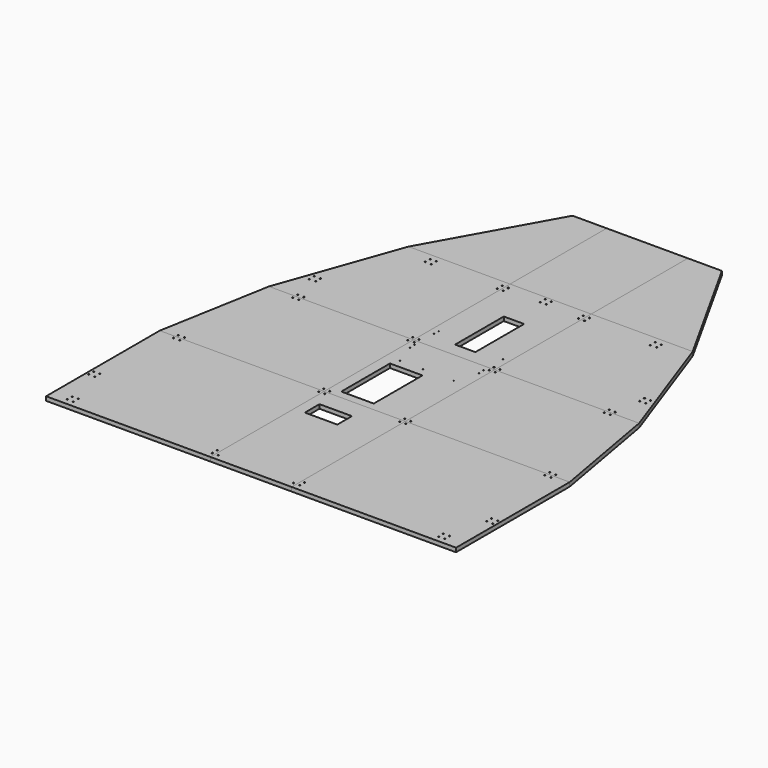
from build123d import *

# Parameters (mm, degrees)
F0_W      = 400
F0_H      = 700
F0_R      = 3
F0_W_2    = 160
F0_H_2    = 89.9538263201
F1_DEPTH  = 20
F2_R      = 3
F3_DEPTH  = 20
F4_DEPTH  = 20
F5_W      = 400
F5_H      = 550
F5_R      = 3
F5_W_2    = 160
F5_H_2    = 300
F5_R_2    = 2.05
F6_DEPTH  = 20
F7_W      = 400
F7_H      = 595
F7_R      = 3
F7_R_2    = 2.05
F7_W_2    = 100
F7_H_2    = 300
F8_DEPTH  = 20
F9_W      = 760
F9_H      = 700
F9_R      = 3
F10_DEPTH = 20
F11_W     = 400
F11_H     = 595
F12_DEPTH = 20
F14_DEPTH = 20
F16_DEPTH = 20
F17_W     = 50
F17_H     = 700
F17_R     = 3
F19_DEPTH = 20
F18_W     = 50
F18_H     = 700
F18_R     = 3
F20_DEPTH = 20
F21_R     = 3
F23_DEPTH = 20
F22_R     = 3
F24_DEPTH = 20
F26_DEPTH = 20
F28_DEPTH = 20
F30_DEPTH = 20
F32_DEPTH = 20


with BuildPart() as f1:
    # F0 (on Top) → F1 (new body)
    with BuildSketch(Plane.XY):
        Rectangle(F0_W, F0_H)
        with Locations((-185, -320)):
            Circle(F0_R, mode=Mode.SUBTRACT)
        with Locations((185, -320)):
            Circle(F0_R, mode=Mode.SUBTRACT)
        with Locations((-185, 335)):
            Circle(F0_R, mode=Mode.SUBTRACT)
        with Locations((-67.5, 210.6490433216)):
            Rectangle(F0_W_2, F0_H_2, mode=Mode.SUBTRACT)
        with Locations((185, 335)):
            Circle(F0_R, mode=Mode.SUBTRACT)
    extrude(amount=F1_DEPTH)


with BuildPart() as f3:
    # F2 (on Top) → F3 (new body)
    with BuildSketch(Plane.XY):
        Polygon((-200, 350), (-200, 900), (-812, 900), (-960, 350), align=None)
        with Locations((-930, 365)):
            Circle(F2_R, mode=Mode.SUBTRACT)
        with Locations((-900, 365)):
            Circle(F2_R, mode=Mode.SUBTRACT)
        with Locations((-215, 365)):
            Circle(F2_R, mode=Mode.SUBTRACT)
        with Locations((-782, 885)):
            Circle(F2_R, mode=Mode.SUBTRACT)
        with Locations((-752, 885)):
            Circle(F2_R, mode=Mode.SUBTRACT)
        with Locations((-215, 885)):
            Circle(F2_R, mode=Mode.SUBTRACT)
    extrude(amount=F3_DEPTH)

    # F25 (on face) → F26 (join)
    with BuildSketch(Plane(origin=(0, 0, 0), x_dir=(1, 0, 0), z_dir=(0, 0, -1))):
        Polygon((-912, -900), (-812, -900), (-960, -350), (-1010, -350), align=None)
    extrude(amount=-F26_DEPTH)


with BuildPart() as f3b:
    # F2 (on Top) → F3, piece 2 (new body)
    with BuildSketch(Plane.XY):
        Polygon((812, 900), (200, 900), (200, 350), (960, 350), align=None)
        with Locations((215, 365)):
            Circle(F2_R, mode=Mode.SUBTRACT)
        with Locations((900, 365)):
            Circle(F2_R, mode=Mode.SUBTRACT)
        with Locations((930, 365)):
            Circle(F2_R, mode=Mode.SUBTRACT)
        with Locations((215, 885)):
            Circle(F2_R, mode=Mode.SUBTRACT)
        with Locations((752, 885)):
            Circle(F2_R, mode=Mode.SUBTRACT)
        with Locations((782, 885)):
            Circle(F2_R, mode=Mode.SUBTRACT)
    extrude(amount=F3_DEPTH)

    # F27 (on face) → F28 (join)
    with BuildSketch(Plane(origin=(0, 0, 0), x_dir=(1, 0, 0), z_dir=(0, 0, -1))):
        Polygon((1010, -350), (960, -350), (812, -900), (912, -900), align=None)
    extrude(amount=-F28_DEPTH)


with BuildPart() as f4:
    # F2 (on Top) → F4 (new body)
    with BuildSketch(Plane.XY):
        Polygon((-812, 900), (-200, 900), (-200, 1495), (-600, 1495), align=None)
        with Locations((-782, 915)):
            Circle(F2_R, mode=Mode.SUBTRACT)
        with Locations((-752, 915)):
            Circle(F2_R, mode=Mode.SUBTRACT)
        with Locations((-215, 915)):
            Circle(F2_R, mode=Mode.SUBTRACT)
        with Locations((-570, 1435)):
            Circle(F2_R, mode=Mode.SUBTRACT)
        with Locations((-540, 1435)):
            Circle(F2_R, mode=Mode.SUBTRACT)
        with Locations((-570, 1465)):
            Circle(F2_R, mode=Mode.SUBTRACT)
        with Locations((-540, 1465)):
            Circle(F2_R, mode=Mode.SUBTRACT)
        with Locations((-215, 1435)):
            Circle(F2_R, mode=Mode.SUBTRACT)
        with Locations((-215, 1465)):
            Circle(F2_R, mode=Mode.SUBTRACT)
    extrude(amount=F4_DEPTH)

    # F21 (on face) → F23 (join)
    with BuildSketch(Plane(origin=(0, 0, 0), x_dir=(1, 0, 0), z_dir=(0, 0, -1))):
        Polygon((-700, -1495), (-600, -1495), (-812, -900), (-912, -900), align=None)
        with Locations((-828.415464569, -1075)):
            Circle(F21_R, mode=Mode.SUBTRACT)
        with Locations((-798.415464569, -1075)):
            Circle(F21_R, mode=Mode.SUBTRACT)
        with Locations((-828.415464569, -1045)):
            Circle(F21_R, mode=Mode.SUBTRACT)
        with Locations((-798.415464569, -1045)):
            Circle(F21_R, mode=Mode.SUBTRACT)
    extrude(amount=-F23_DEPTH)


with BuildPart() as f4b:
    # F2 (on Top) → F4, piece 2 (new body)
    with BuildSketch(Plane.XY):
        Polygon((600, 1495), (200, 1495), (200, 900), (812, 900), align=None)
        with Locations((215, 915)):
            Circle(F2_R, mode=Mode.SUBTRACT)
        with Locations((752, 915)):
            Circle(F2_R, mode=Mode.SUBTRACT)
        with Locations((782, 915)):
            Circle(F2_R, mode=Mode.SUBTRACT)
        with Locations((215, 1435)):
            Circle(F2_R, mode=Mode.SUBTRACT)
        with Locations((215, 1465)):
            Circle(F2_R, mode=Mode.SUBTRACT)
        with Locations((540, 1435)):
            Circle(F2_R, mode=Mode.SUBTRACT)
        with Locations((570, 1435)):
            Circle(F2_R, mode=Mode.SUBTRACT)
        with Locations((540, 1465)):
            Circle(F2_R, mode=Mode.SUBTRACT)
        with Locations((570, 1465)):
            Circle(F2_R, mode=Mode.SUBTRACT)
    extrude(amount=F4_DEPTH)

    # F22 (on face) → F24 (join)
    with BuildSketch(Plane(origin=(0, 0, 0), x_dir=(1, 0, 0), z_dir=(0, 0, -1))):
        Polygon((912, -900), (812, -900), (600, -1495), (700, -1495), align=None)
        with Locations((798.415464569, -1075)):
            Circle(F22_R, mode=Mode.SUBTRACT)
        with Locations((828.415464569, -1075)):
            Circle(F22_R, mode=Mode.SUBTRACT)
        with Locations((798.415464569, -1045)):
            Circle(F22_R, mode=Mode.SUBTRACT)
        with Locations((828.415464569, -1045)):
            Circle(F22_R, mode=Mode.SUBTRACT)
    extrude(amount=-F24_DEPTH)


with BuildPart() as f6:
    # F5 (on Top) → F6 (new body)
    with BuildSketch(Plane.XY):
        with Locations((0, 625)):
            Rectangle(F5_W, F5_H)
        with Locations((-185, 365)):
            Circle(F5_R, mode=Mode.SUBTRACT)
        with Locations((-67.5, 540)):
            Rectangle(F5_W_2, F5_H_2, mode=Mode.SUBTRACT)
        with Locations((185, 365)):
            Circle(F5_R, mode=Mode.SUBTRACT)
        with Locations((-132.5, 731.5)):
            Circle(F5_R_2, mode=Mode.SUBTRACT)
        with Locations((-17.5, 731.5)):
            Circle(F5_R_2, mode=Mode.SUBTRACT)
        with Locations((-170, 840)):
            Circle(F5_R_2, mode=Mode.SUBTRACT)
        with Locations((-185, 885)):
            Circle(F5_R, mode=Mode.SUBTRACT)
        with Locations((-170, 870)):
            Circle(F5_R_2, mode=Mode.SUBTRACT)
        with Locations((132.5, 731.5)):
            Circle(F5_R_2, mode=Mode.SUBTRACT)
        with Locations((170, 840)):
            Circle(F5_R_2, mode=Mode.SUBTRACT)
        with Locations((170, 870)):
            Circle(F5_R_2, mode=Mode.SUBTRACT)
        with Locations((185, 885)):
            Circle(F5_R, mode=Mode.SUBTRACT)
    extrude(amount=F6_DEPTH)


with BuildPart() as f8:
    # F7 (on Top) → F8 (new body)
    with BuildSketch(Plane.XY):
        with Locations((0, 1197.5)):
            Rectangle(F7_W, F7_H)
        with Locations((-185, 915)):
            Circle(F7_R, mode=Mode.SUBTRACT)
        with Locations((-170, 988)):
            Circle(F7_R_2, mode=Mode.SUBTRACT)
        with Locations((-170, 1018)):
            Circle(F7_R_2, mode=Mode.SUBTRACT)
        with Locations((185, 915)):
            Circle(F7_R, mode=Mode.SUBTRACT)
        with Locations((170, 988)):
            Circle(F7_R_2, mode=Mode.SUBTRACT)
        with Locations((170, 1018)):
            Circle(F7_R_2, mode=Mode.SUBTRACT)
        with Locations((0, 1119.0668344498)):
            Rectangle(F7_W_2, F7_H_2, mode=Mode.SUBTRACT)
        with Locations((-185, 1435)):
            Circle(F7_R, mode=Mode.SUBTRACT)
        with Locations((-185, 1465)):
            Circle(F7_R, mode=Mode.SUBTRACT)
        with Locations((-15, 1450)):
            Circle(F7_R, mode=Mode.SUBTRACT)
        with Locations((-15, 1480)):
            Circle(F7_R, mode=Mode.SUBTRACT)
        with Locations((15, 1450)):
            Circle(F7_R, mode=Mode.SUBTRACT)
        with Locations((15, 1480)):
            Circle(F7_R, mode=Mode.SUBTRACT)
        with Locations((185, 1435)):
            Circle(F7_R, mode=Mode.SUBTRACT)
        with Locations((185, 1465)):
            Circle(F7_R, mode=Mode.SUBTRACT)
    extrude(amount=F8_DEPTH)


with BuildPart() as f10:
    # F9 (on Top) → F10 (new body)
    with BuildSketch(Plane.XY):
        with Locations((-580, 0)):
            Rectangle(F9_W, F9_H)
        with Locations((-930, -320)):
            Circle(F9_R, mode=Mode.SUBTRACT)
        with Locations((-900, -320)):
            Circle(F9_R, mode=Mode.SUBTRACT)
        with Locations((-930, -290)):
            Circle(F9_R, mode=Mode.SUBTRACT)
        with Locations((-900, -290)):
            Circle(F9_R, mode=Mode.SUBTRACT)
        with Locations((-215, -320)):
            Circle(F9_R, mode=Mode.SUBTRACT)
        with Locations((-215, -290)):
            Circle(F9_R, mode=Mode.SUBTRACT)
        with Locations((-930, 335)):
            Circle(F9_R, mode=Mode.SUBTRACT)
        with Locations((-900, 335)):
            Circle(F9_R, mode=Mode.SUBTRACT)
        with Locations((-215, 335)):
            Circle(F9_R, mode=Mode.SUBTRACT)
    extrude(amount=F10_DEPTH)

    # F17 (on face) → F19 (join)
    with BuildSketch(Plane(origin=(0, 0, 0), x_dir=(1, 0, 0), z_dir=(0, 0, -1))):
        with Locations((-985, 0)):
            Rectangle(F17_W, F17_H)
        with Locations((-995, 75)):
            Circle(F17_R, mode=Mode.SUBTRACT)
        with Locations((-995, 105)):
            Circle(F17_R, mode=Mode.SUBTRACT)
        with Locations((-965, 75)):
            Circle(F17_R, mode=Mode.SUBTRACT)
        with Locations((-965, 105)):
            Circle(F17_R, mode=Mode.SUBTRACT)
    extrude(amount=-F19_DEPTH)


with BuildPart() as f10b:
    # F9 (on Top) → F10, piece 2 (new body)
    with BuildSketch(Plane.XY):
        with Locations((580, 0)):
            Rectangle(F9_W, F9_H)
        with Locations((215, -320)):
            Circle(F9_R, mode=Mode.SUBTRACT)
        with Locations((215, -290)):
            Circle(F9_R, mode=Mode.SUBTRACT)
        with Locations((900, -320)):
            Circle(F9_R, mode=Mode.SUBTRACT)
        with Locations((930, -320)):
            Circle(F9_R, mode=Mode.SUBTRACT)
        with Locations((900, -290)):
            Circle(F9_R, mode=Mode.SUBTRACT)
        with Locations((930, -290)):
            Circle(F9_R, mode=Mode.SUBTRACT)
        with Locations((215, 335)):
            Circle(F9_R, mode=Mode.SUBTRACT)
        with Locations((900, 335)):
            Circle(F9_R, mode=Mode.SUBTRACT)
        with Locations((930, 335)):
            Circle(F9_R, mode=Mode.SUBTRACT)
    extrude(amount=F10_DEPTH)

    # F18 (on face) → F20 (join)
    with BuildSketch(Plane(origin=(0, 0, 0), x_dir=(1, 0, 0), z_dir=(0, 0, -1))):
        with Locations((985, 0)):
            Rectangle(F18_W, F18_H)
        with Locations((965, 75)):
            Circle(F18_R, mode=Mode.SUBTRACT)
        with Locations((965, 105)):
            Circle(F18_R, mode=Mode.SUBTRACT)
        with Locations((995, 75)):
            Circle(F18_R, mode=Mode.SUBTRACT)
        with Locations((995, 105)):
            Circle(F18_R, mode=Mode.SUBTRACT)
    extrude(amount=-F20_DEPTH)


with BuildPart() as f12:
    # F11 (on face) → F12 (new body)
    with BuildSketch(Plane.XY.offset(20)):
        with Locations((0, 1792.5)):
            Rectangle(F11_W, F11_H)
    extrude(amount=-F12_DEPTH)


with BuildPart() as f14:
    # F13 (on face) → F14 (new body)
    with BuildSketch(Plane.XY.offset(20)):
        Polygon((-600, 1495), (-200, 1495), (-200, 2090), (-268, 2090), align=None)
    extrude(amount=-F14_DEPTH)

    # F31 (on face) → F32 (join)
    with BuildSketch(Plane(origin=(0, 0, 0), x_dir=(1, 0, 0), z_dir=(0, 0, -1))):
        Polygon((-268, -2090), (-600, -1495), (-700, -1495), (-368, -2090), align=None)
    extrude(amount=-F32_DEPTH)


with BuildPart() as f16:
    # F15 (on face) → F16 (new body)
    with BuildSketch(Plane.XY.offset(20)):
        Polygon((200, 2090), (200, 1495), (600, 1495), (268, 2090), align=None)
    extrude(amount=-F16_DEPTH)

    # F29 (on face) → F30 (join)
    with BuildSketch(Plane(origin=(0, 0, 0), x_dir=(1, 0, 0), z_dir=(0, 0, -1))):
        Polygon((700, -1495), (600, -1495), (268, -2090), (368, -2090), align=None)
    extrude(amount=-F30_DEPTH)


solid = Compound([f1.part, f3.part, f3b.part, f4.part, f4b.part, f6.part, f8.part, f10.part, f10b.part, f12.part, f14.part, f16.part])
